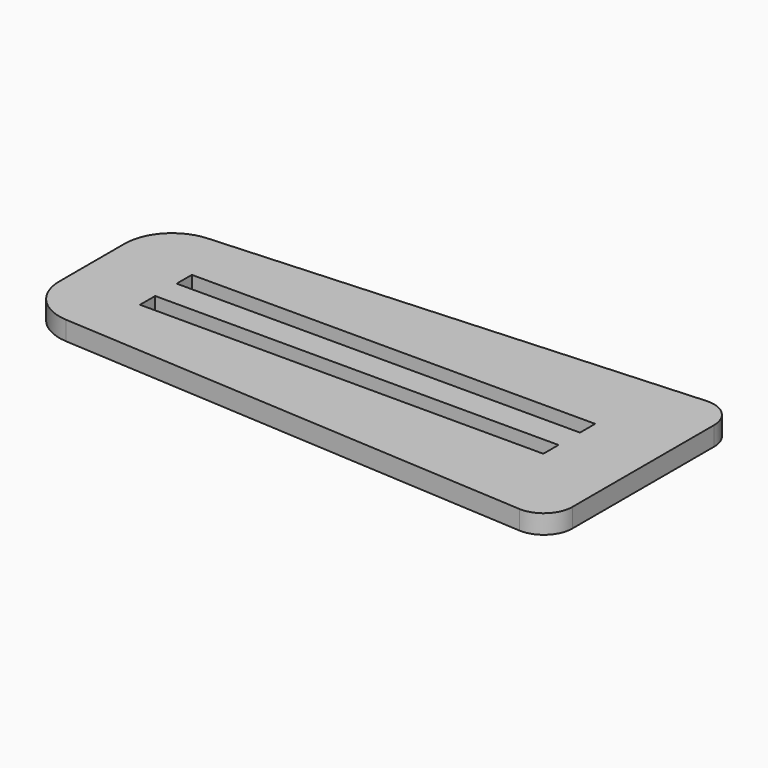
from build123d import *

# Parameters (mm, degrees)
F0_W     = 42.4481438452
F0_H     = 2
F1_DEPTH = 2
F2_R     = 3
F3_R     = 5


with BuildPart() as f1:
    # F0 (on Top) → F1 (new body)
    with BuildSketch(Plane.XY):
        Polygon((-65.7136544558, 44.0634722376), (-65.7136544558, 36.4734722376), (-65.7136544558, 35.0634722376), (-65.7136544558, 33.6534722376), (-65.7136544558, 26.0634722376), (-7.7136544558, 22.5634722376), (-7.7136544558, 47.5634722376), align=None)
        with Locations((-36.7136544558, 32.6534722376)):
            Rectangle(F0_W, F0_H, mode=Mode.SUBTRACT)
        with Locations((-36.7136544558, 37.4734722376)):
            Rectangle(F0_W, F0_H, mode=Mode.SUBTRACT)
    extrude(amount=F1_DEPTH)

    # F2
    f2_edges = [f1.edges().sort_by_distance(p)[0] for p in [
        (-7.713654, 47.563472, 1),
        (-7.713654, 22.563472, 1),
    ]]
    fillet(f2_edges, radius=F2_R)

    # F3
    f3_edges = [f1.edges().sort_by_distance(p)[0] for p in [
        (-65.713654, 26.063472, 1),
        (-65.713654, 44.063472, 1),
    ]]
    fillet(f3_edges, radius=F3_R)


solid = f1.part
